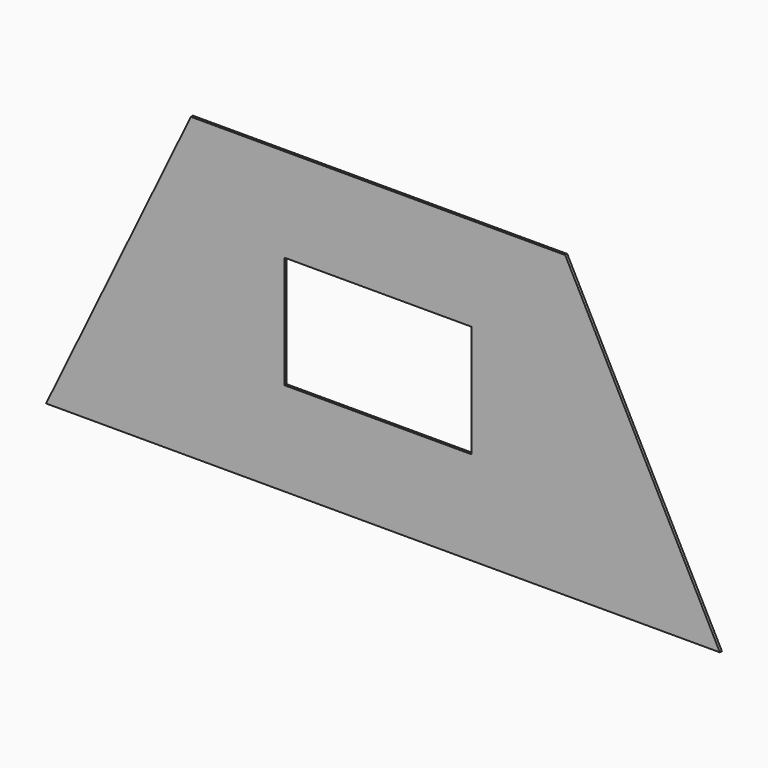
from build123d import *

# Parameters (mm, degrees)
F0_W     = 254
F0_H     = 152.4
F1_DEPTH = 3.4036


# Not quite as in the source:
# - a feature names something its author has since deleted; it is built from what else it names


with BuildPart() as f1:
    # F0 (on Front) → F1 (new body)
    with BuildSketch(Plane.XZ):
        Polygon((196.4755472482, 406.4), (0, 0), (914.4, 0), (704.4755472482, 406.4), align=None)
        with Locations((450.4755472482, 203.2)):
            Rectangle(F0_W, F0_H, mode=Mode.SUBTRACT)
    extrude(amount=F1_DEPTH)


solid = f1.part
